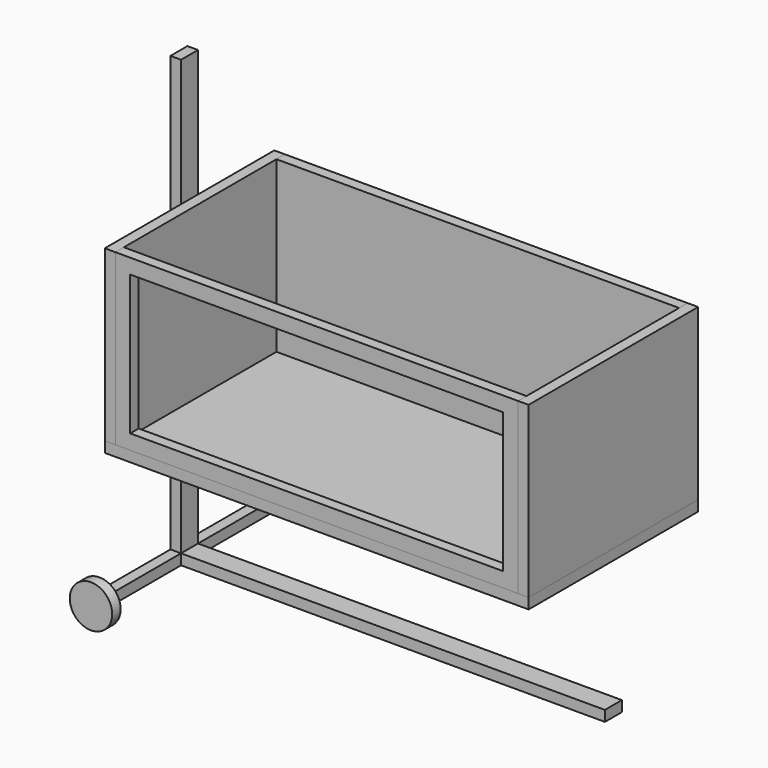
from build123d import *

# Parameters (mm, degrees)
F0_W           = 1000
F0_H           = 500
F1_DEPTH       = 25
F2_W           = 25
F2_H           = 500
F3_DEPTH       = 400
F4_W           = 25
F4_H           = 500
F5_DEPTH       = 400
F6_W           = 950
F6_H           = 25
F7_DEPTH       = 400
F8_W           = 950
F8_H           = 25
F9_DEPTH       = 400
F10_W          = 50
F10_H          = 1025
F11_DEPTH      = 25
F12_W          = 50
F12_H          = 1025
F13_DEPTH      = 25
F14_W          = 1000
F14_H          = 50
F15_DEPTH      = 25
F16_W          = 25
F16_H          = 25
F17_DEPTH      = 250
F17_DEPTH_BACK = 250
F18_R          = 50
F19_DEPTH      = 25
F21_W          = 880
F21_H          = 330
F22_DEPTH      = 500.001


# Not quite as in the source:
# - the program builds the solid bodies; features that only make, move or delete a surface that nothing else refers to are left out


with BuildPart() as f1:
    # F0 (on Top) → F1 (new body)
    with BuildSketch(Plane.XY):
        Rectangle(F0_W, F0_H)
    extrude(amount=F1_DEPTH)


with BuildPart() as f3:
    # F2 (on face) → F3 (new body)
    with BuildSketch(Plane.XY.offset(25)):
        with Locations((-487.5, 0)):
            Rectangle(F2_W, F2_H)
    extrude(amount=F3_DEPTH)


with BuildPart() as f5:
    # F4 (on face) → F5 (new body, through all)
    with BuildSketch(Plane.XY.offset(25)):
        with Locations((487.5, 0)):
            Rectangle(F4_W, F4_H)
    extrude(amount=F5_DEPTH)


with BuildPart() as f7:
    # F6 (on face) → F7 (new body, through all)
    with BuildSketch(Plane.XY.offset(25)):
        with Locations((0, 237.5)):
            Rectangle(F6_W, F6_H)
    extrude(amount=F7_DEPTH)


with BuildPart() as f9:
    # F8 (on face) → F9 (new body, through all)
    with BuildSketch(Plane.XY.offset(25)):
        with Locations((0, -237.5)):
            Rectangle(F8_W, F8_H)
    extrude(amount=F9_DEPTH)

    # F21 (on face) → F22 (cut, through all)
    with BuildSketch(Plane.XZ.offset(250)):
        with Locations((0, 225)):
            Rectangle(F21_W, F21_H)
    extrude(amount=-F22_DEPTH, mode=Mode.SUBTRACT)


with BuildPart() as f11:
    # F10 (on face) → F11 (new body)
    with BuildSketch(Plane.YZ.offset(500)):
        with Locations((0, 212.5)):
            Rectangle(F10_W, F10_H)
    extrude(amount=F11_DEPTH)


with BuildPart() as f13:
    # F12 (on face) → F13 (new body)
    with BuildSketch(Plane(origin=(-500, 0, 0), x_dir=(0, -1, 0), z_dir=(-1, 0, 0))):
        with Locations((0, 212.5)):
            Rectangle(F12_W, F12_H)
    extrude(amount=F13_DEPTH)


with BuildPart() as f15:
    # F14 (on face) → F15 (new body)
    with BuildSketch(Plane(origin=(0, 0, -300), x_dir=(1, 0, 0), z_dir=(0, 0, -1))):
        Rectangle(F14_W, F14_H)
    extrude(amount=F15_DEPTH)


with BuildPart() as f17:
    # F16 (on Front) → F17 (new body, two sides)
    with BuildSketch(Plane.XZ) as f17_sk:
        with Locations((-512.5, -312.5)):
            Rectangle(F16_W, F16_H)
    extrude(amount=F17_DEPTH)
    extrude(f17_sk.sketch, amount=-F17_DEPTH_BACK)


with BuildPart() as f19:
    # F18 (on face) → F19 (new body)
    with BuildSketch(Plane.XZ.offset(250)):
        with Locations((-512.5, -312.5)):
            Circle(F18_R)
    extrude(amount=F19_DEPTH)


solid = Compound([f1.part, f3.part, f5.part, f7.part, f9.part, f13.part, f15.part, f17.part, f19.part])
